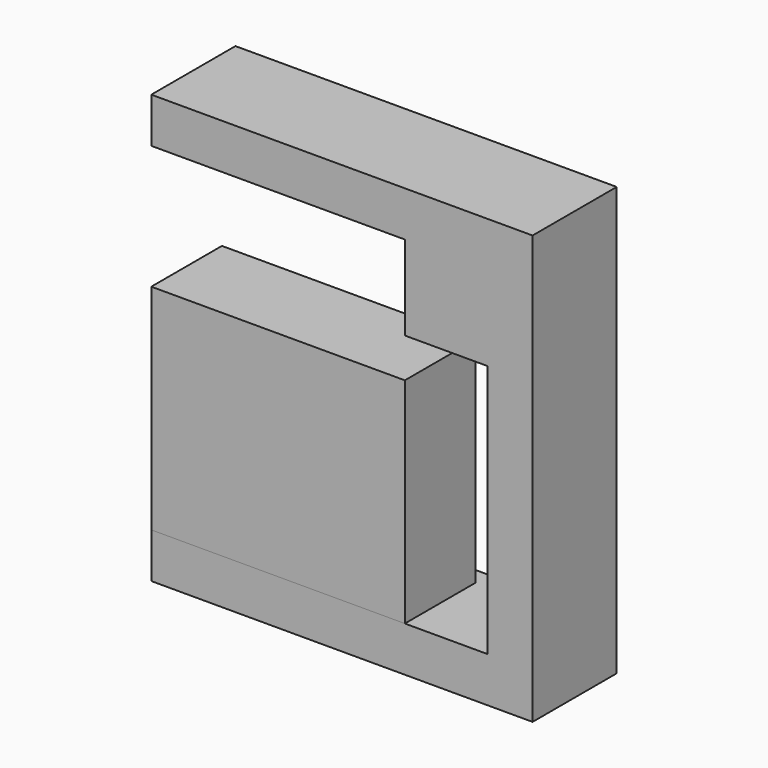
from build123d import *

# Parameters (mm, degrees)
F1_DEPTH = 355.6
F2_W     = 1714.5
F2_H     = 1447.8
F3_DEPTH = 355.6
F4_W     = 1714.5
F4_H     = 1447.8
F5_DEPTH = 241.3


# Not quite as in the source:
# - a length typed as a fraction of an inch, garbled in the dataset ("3 / 203.2 mm" for 3/8 in), is restored


with BuildPart() as f1:
    # F0 (on Front) → F1 (new body, symmetric)
    with BuildSketch(Plane.XZ):
        Polygon((1136.65, 1714.5), (1136.65, 0), (-1136.65, 0), (-1136.65, -304.8), (1441.45, -304.8), (1441.45, 2590.8), (-1136.65, 2590.8), (-1136.65, 2286), (577.85, 2286), (577.85, 1714.5), align=None)
    extrude(amount=F1_DEPTH, both=True)


with BuildPart() as f3:
    # F2 (on Front) → F3 (new body)
    with BuildSketch(Plane.XZ):
        with Locations((-279.4, 723.9)):
            Rectangle(F2_W, F2_H)
    extrude(amount=F3_DEPTH)

    # F4 (on face) → F5 (join)
    with BuildSketch(Plane(origin=(0, 0, 0), x_dir=(-1, 0, 0), z_dir=(0, 1, 0))):
        with Locations((279.4, 723.9)):
            Rectangle(F4_W, F4_H)
    extrude(amount=F5_DEPTH)


solid = Compound([f1.part, f3.part])
